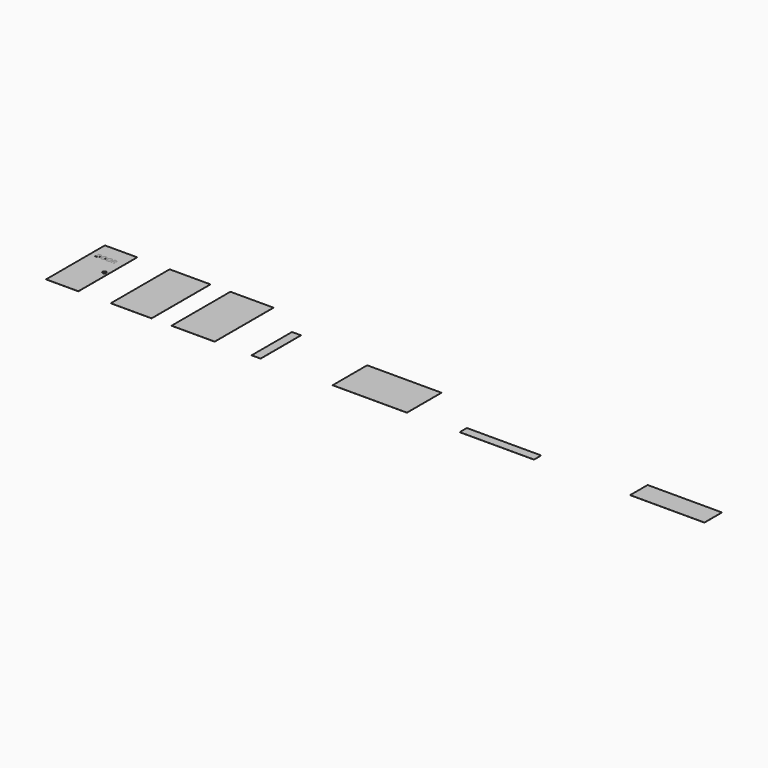
from build123d import *

# Parameters (mm, degrees)
F0_W         = 850
F0_H         = 1936
F0_R         = 47.4152483598
F1_DEPTH     = 2
F0_W_2       = 1074
F0_W_3       = 1136
F0_W_4       = 236
F0_H_2       = 1328
F0_W_5       = 1956
F0_H_3       = 1136
F0_H_4       = 236
F0_H_5       = 576
F2_TEXT_SIZE = 183.5372712877
F3_DEPTH     = 1


# Not quite as in the source:
# - Text() gives the source's letters only with a copy of the font that has no kerning and outlines rounded to 1/6400 em; it was checked with that copy


with BuildPart() as f1:
    # F0 (on Top) → F1 (new body)
    with BuildSketch(Plane.XY):
        with Locations((-425, 968)):
            Rectangle(F0_W, F0_H)
        with Locations((-108.9282333851, 992.445230484)):
            Circle(F0_R, mode=Mode.SUBTRACT)
    extrude(amount=F1_DEPTH)

    # F2 (on face) → F3 (cut)
    with BuildSketch(Plane.XY.offset(2)):
        with Locations((-721.7562198639, 1422.9583740234)):
            Text('DOOR', F2_TEXT_SIZE, font='Open Sans', text_align=(TextAlign.LEFT, TextAlign.BOTTOM))
    extrude(amount=-F3_DEPTH, mode=Mode.SUBTRACT)


with BuildPart() as f1b:
    # F0 (on Top) → F1, piece 2 (new body)
    with BuildSketch(Plane.XY):
        with Locations((1390.9797663689, 968)):
            Rectangle(F0_W_2, F0_H)
    extrude(amount=F1_DEPTH)


with BuildPart() as f1c:
    # F0 (on Top) → F1, piece 3 (new body)
    with BuildSketch(Plane.XY):
        with Locations((3021.8750648499, 968)):
            Rectangle(F0_W_3, F0_H)
    extrude(amount=F1_DEPTH)


with BuildPart() as f1d:
    # F0 (on Top) → F1, piece 4 (new body)
    with BuildSketch(Plane.XY):
        with Locations((4680.8280639648, 664)):
            Rectangle(F0_W_4, F0_H_2)
    extrude(amount=F1_DEPTH)


with BuildPart() as f1e:
    # F0 (on Top) → F1, piece 5 (new body)
    with BuildSketch(Plane.XY):
        with Locations((7673.8632469177, 568)):
            Rectangle(F0_W_5, F0_H_3)
    extrude(amount=F1_DEPTH)


with BuildPart() as f1f:
    # F0 (on Top) → F1, piece 6 (new body)
    with BuildSketch(Plane.XY):
        with Locations((11019.0985946655, 118)):
            Rectangle(F0_W_5, F0_H_4)
    extrude(amount=F1_DEPTH)


with BuildPart() as f1g:
    # F0 (on Top) → F1, piece 7 (new body)
    with BuildSketch(Plane.XY):
        with Locations((15507.1166305542, 288)):
            Rectangle(F0_W_5, F0_H_5)
    extrude(amount=F1_DEPTH)


solid = Compound([f1.part, f1b.part, f1c.part, f1d.part, f1e.part, f1f.part, f1g.part])
